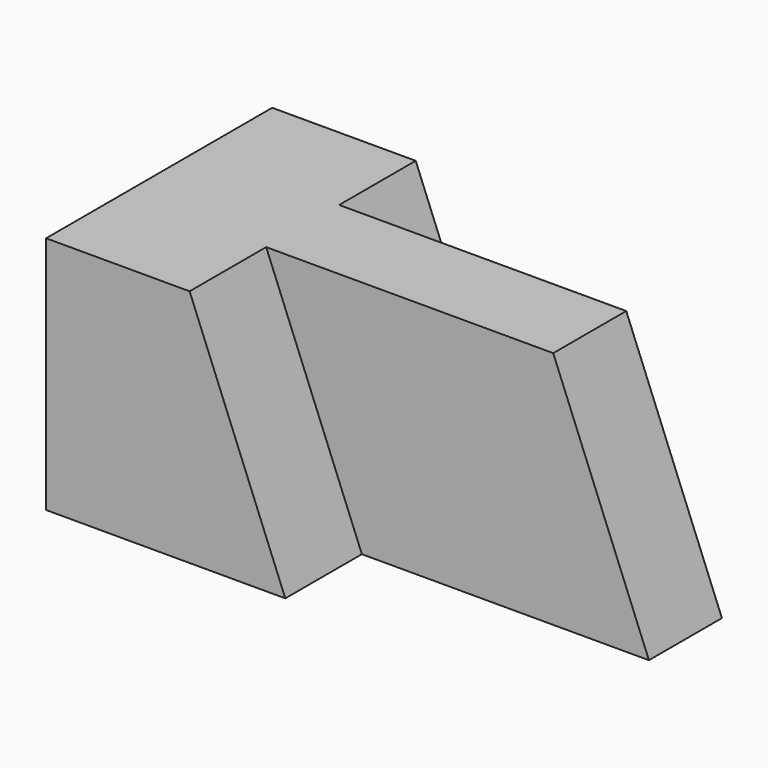
from build123d import *

# Parameters (mm, degrees)
F1_DEPTH = 31.75
F3_DEPTH = 25.4
F5_DEPTH = 12.7
F7_DEPTH = 12.7
F8_DEPTH = 25.4


with BuildPart() as f1:
    # F0 (on Top) → F1 (new body)
    with BuildSketch(Plane.XY):
        Polygon((0, 37.5093027622), (0, 0), (31.75, 0), (31.75, 12.7), (69.85, 12.7), (69.85, 24.8093027622), (31.75, 24.8093027622), (31.75, 37.5093027622), align=None)
    extrude(amount=F1_DEPTH)

    # F2 (on face) → F3 (cut)
    with BuildSketch(Plane.XZ.offset(-12.7)):
        Polygon((57.15, 31.75), (69.85, 0), (69.85, 31.75), align=None)
    extrude(amount=-F3_DEPTH, mode=Mode.SUBTRACT)

    # F4 (on face) → F5 (cut)
    with BuildSketch(Plane.XZ):
        Polygon((19.05, 31.75), (31.75, 0), (31.75, 31.75), align=None)
    extrude(amount=-F5_DEPTH, mode=Mode.SUBTRACT)

    # F6 (on face) → F7 (join)
    with BuildSketch(Plane(origin=(0, 37.5093027622, 0), x_dir=(-1, 0, 0), z_dir=(0, 1, 0))):
        Polygon((-31.75, 31.75), (-31.75, 0), (-19.05, 31.75), align=None)
    extrude(amount=F7_DEPTH)

    # F8 (cut): a face of the model
    f8_faces = [f1.faces().sort_by_distance(p)[0] for p in [
        (27.5166666667, 50.2093027622, 21.1666666667),
    ]]
    extrude(f8_faces, amount=-F8_DEPTH, mode=Mode.SUBTRACT)


solid = f1.part
